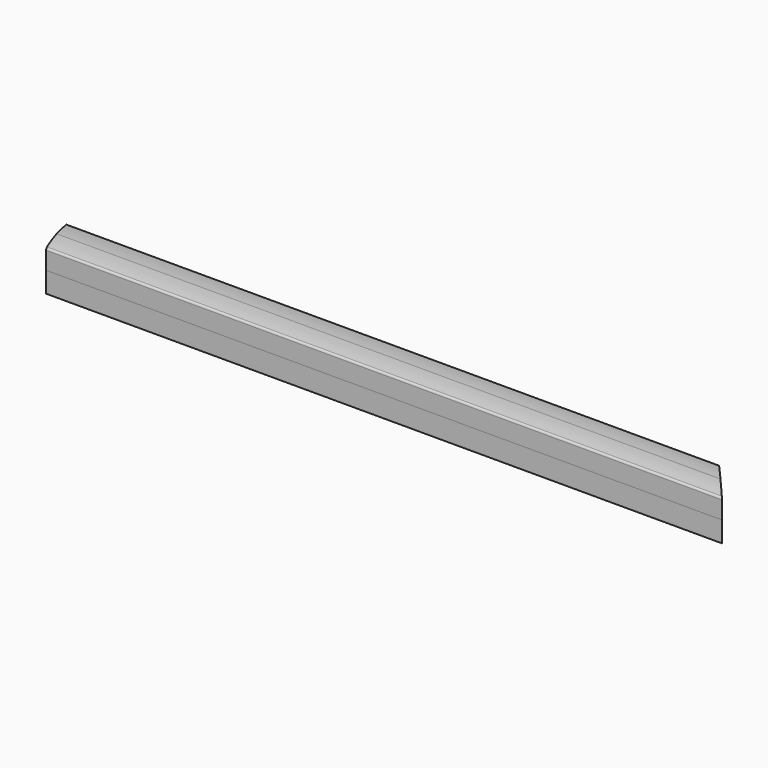
from build123d import *

# Parameters (mm, degrees)
F2_DEPTH      = 1000
F4_DEPTH      = 1000
F8_DEPTH      = 10.001
F8_DEPTH_BACK = 10.001


with BuildPart() as f2:
    # F1 (on Right) → F2 (new body)
    with BuildSketch(Plane.YZ):
        with BuildLine():
            Line((0, -9), (0, -10))
            Line((0, -10), (10, -10))
            Line((10, -10), (10, -0.2))
            Line((10, -0.2), (9, -0.2))
            ThreePointArc((9, -0.2), (8.5, -0.7), (9, -1.2))
            ThreePointArc((9, -1.2), (9.5, -1.7), (9, -2.2))
            Line((9, -2.2), (9, -9))
            Line((9, -9), (0, -9))
        make_face()
    extrude(amount=F2_DEPTH)

    # F5: F2 across plane


with BuildPart() as f4:
    # F3 (on Right) → F4 (new body)
    with BuildSketch(Plane.YZ):
        with BuildLine():
            Line((9, -0.2), (10, -0.2))
            Line((10, -0.2), (10, 8.1663783152))
            ThreePointArc((10, 8.1663783152), (9.7693092582, 8.8052548802), (9.1836734694, 9.1493656277))
            ThreePointArc((9.1836734694, 9.1493656277), (4.6114920912, 9.7868872364), (0, 10))
            Line((0, 10), (0, 9))
            ThreePointArc((0, 9), (4.5192622493, 8.7911494917), (9, 8.1663783152))
            Line((9, 8.1663783152), (9, 0.8))
            ThreePointArc((9, 0.8), (7.5, -0.7), (9, -2.2))
            ThreePointArc((9, -2.2), (9.5, -1.7), (9, -1.2))
            ThreePointArc((9, -1.2), (8.5, -0.7), (9, -0.2))
        make_face()
    extrude(amount=F4_DEPTH)

    # F6: F4 across plane


with BuildPart() as f2_1:
    add(f2.part)
    add(f2.part.mirror(Plane.XZ))


with BuildPart() as f4_1:
    add(f4.part)
    add(f4.part.mirror(Plane.XZ))


with BuildPart() as f8_tool:
    # F7 (on Top) → F8 (new body, two sides)
    with BuildSketch(Plane.XY) as f8_sk:
        Polygon((0, 10), (0, 0), (0, -10), (6.0383560074, -10), align=None)
        Polygon((709.9114181152, 10), (309.652621251, 10), (327.0383560074, -10), (1016.9613361359, -10), (1016.9613361359, 10), align=None)
    extrude(amount=F8_DEPTH)
    extrude(f8_sk.sketch, amount=-F8_DEPTH_BACK)


with BuildPart() as f2_2:
    add(f2_1.part)

    # F8: cut by f8_tool
    add(f8_tool.part, mode=Mode.SUBTRACT)


with BuildPart() as f4_2:
    add(f4_1.part)

    # F8: cut by f8_tool
    add(f8_tool.part, mode=Mode.SUBTRACT)


solid = Compound([f2_2.part, f4_2.part])
